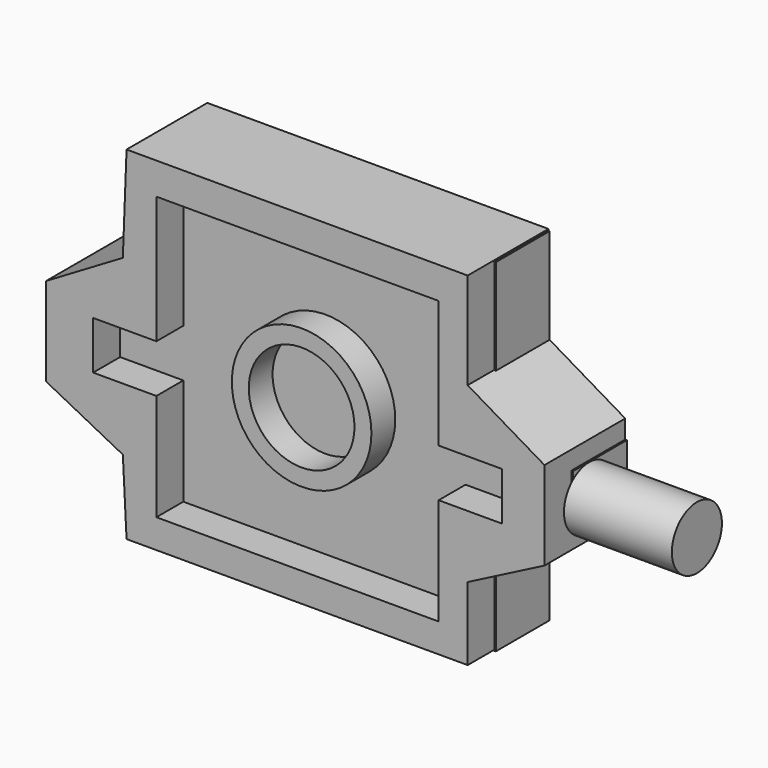
from build123d import *

# Parameters (mm, degrees)
F1_DEPTH = 3.12
F2_R     = 2.44
F3_DEPTH = 1.5
F5_DEPTH = 4.68
F6_R     = 3.235
F6_R_2   = 2.45
F7_DEPTH = 4.5
F9_DEPTH = 5


# Not quite as in the source:
# - the program builds the solid bodies; features that only make, move or delete a surface that nothing else refers to are left out


with BuildPart() as f1:
    # F0 (on Front) → F1 (new body)
    with BuildSketch(Plane.XZ):
        Polygon((14.9867535406, 12.4322535499), (-0.8932464594, 12.4322535499), (-0.8932464594, 5.6322535499), (-0.8932464594, 5.0706164911), (-3.7561513018, 5.0706164911), (-3.7561513018, 2.860605251), (-0.8932464594, 2.860605251), (-0.8932464594, -3.4477464501), (14.9867535406, -3.4477464501), (14.9867535406, 2.860605251), (18.5687988997, 2.860605251), (18.5687988997, 5.0706164911), (14.9867535406, 5.0706164911), (14.9867535406, 5.5522535499), align=None)
    extrude(amount=F1_DEPTH)

    # F2 (on Front) → F3 (join)
    with BuildSketch(Plane.XZ):
        with Locations((11.2367535406, 8.6822535499)):
            Circle(F2_R)
        with Locations((3.1867535406, 8.6822535499)):
            Circle(F2_R)
        with Locations((3.1867535406, 0.6322535499)):
            Circle(F2_R)
        with Locations((11.2367535406, 0.6322535499)):
            Circle(F2_R)
    extrude(amount=-F3_DEPTH)

    # F4 (on Front) → F5 (join)
    with BuildSketch(Plane.XZ):
        Polygon((0.5067535406, 5.13), (0.5067535406, 11.0322535499), (13.5867535406, 11.0322535499), (13.5867535406, 5.13), (14.9343172088, 5.13), (14.9343172088, 8.03), (14.9343172088, 12.5052658841), (-0.8757988689, 12.5052658841), (-1.0476475582, 8.03), (-4.6052209849, 5.9285708389), (-4.6052209849, 1.8285708389), (-1.0476475582, 0), (-0.8757988689, -3.3894693479), (14.9343172088, -3.3894693479), (14.9343172088, 0), (14.9343172088, 2.9), (13.5867535406, 2.9), (13.5867535406, -2.0477464501), (0.5067535406, -2.0477464501), (0.5067535406, 2.9), (-2.4232464594, 2.9), (-2.4232464594, 5.13), align=None)
        Polygon((14.9343172088, 8.03), (14.9343172088, 5.13), (16.5167535406, 5.13), (16.5167535406, 2.9), (14.9343172088, 2.9), (14.9343172088, 0), (18.4918906356, 1.8285708389), (18.4918906356, 5.9285708389), align=None)
    extrude(amount=F5_DEPTH)

    # F6 (on Front) → F7 (join)
    with BuildSketch(Plane.XZ):
        with Locations((7.094095153, 4.4974250309)):
            Circle(F6_R)
        with Locations((7.094095153, 4.4974250309)):
            Circle(F6_R_2, mode=Mode.SUBTRACT)
    extrude(amount=F7_DEPTH)

    # F8 (on face) → F9 (join)
    with BuildSketch(Plane.YZ.offset(18.5687988997)):
        with BuildLine():
            ThreePointArc((-0.7456844895, 3.608182552), (-0.8395787407, 4.1214828522), (-1.1091013145, 4.5683059836))
            Line((-1.1091013145, 4.5683059836), (-3.2822676645, 2.6480591205))
            ThreePointArc((-3.2822676645, 2.6480591205), (-1.6823841893, 2.2520768032), (-0.7456844895, 3.608182552))
        make_face()
        with BuildLine():
            Line((-3.2822676645, 2.6480591205), (-1.1091013145, 4.5683059836))
            ThreePointArc((-1.1091013145, 4.5683059836), (-3.1558079211, 4.694765727), (-3.2822676645, 2.6480591205))
        make_face()
    extrude(amount=F9_DEPTH)


solid = f1.part
